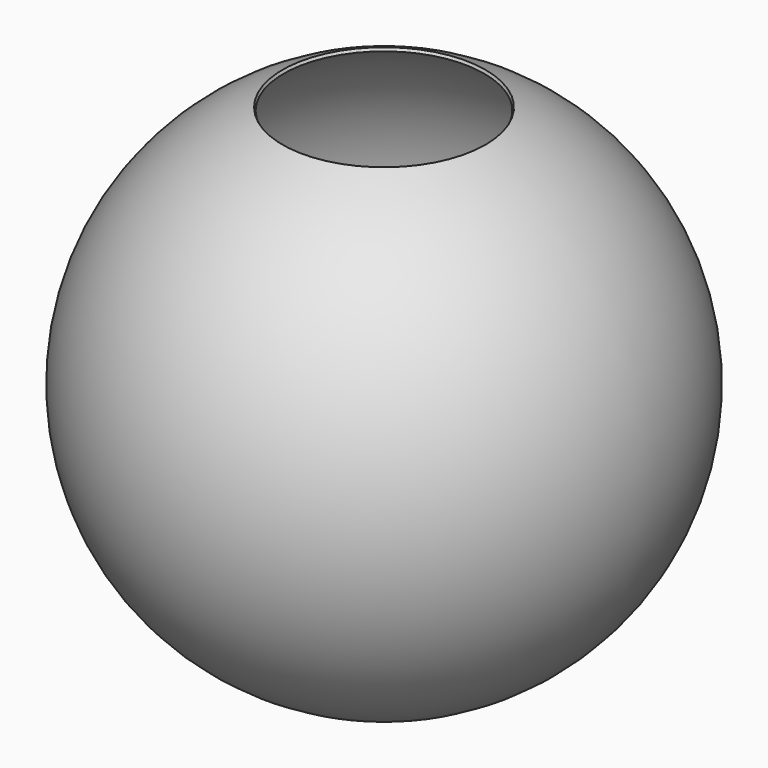
from build123d import *

# Parameters (mm, degrees)
F0_R            = 24
F0_R_2          = 14
F1_DEPTH        = 8
F3_DEPTH        = 1.5
F3_COPIES_COUNT = 5


# Not quite as in the source:
# - a pattern or mirror of a feature is missing from the dataset's text; its kind, count and spacing are read off the source's solid


with BuildPart() as f1:
    # F0 (on Top) → F1 (new body)
    with BuildSketch(Plane.XY):
        Circle(F0_R)
        Circle(F0_R_2, mode=Mode.SUBTRACT)
    extrude(amount=F1_DEPTH)

    # F2 (on Front) → F3 (join, symmetric)
    with BuildSketch(Plane.XZ):
        with BuildLine():
            ThreePointArc((-45.4759894192, -16.4428076923), (-35.9063036344, -5.7161120336), (-22.7166505307, 0))
            Line((-22.7166505307, 0), (-22.7166505307, 8))
            ThreePointArc((-22.7166505307, 8), (-46.7930344517, 15.9905951618), (-64.8907626734, 33.7668182409))
            ThreePointArc((-64.8907626734, 33.7668182409), (-60.6255443353, 6.5576585205), (-45.4759894192, -16.4428076923))
        make_face()
    f3 = extrude(amount=F3_DEPTH, both=True)

    # F3_copies: F3 ×5 about axis
    f3_copies_axis = Axis((0, 0, 0), (0, 0, 1))
    for i in range(1, F3_COPIES_COUNT):
        add(f3.rotate(f3_copies_axis, i * 360 / F3_COPIES_COUNT))


with BuildPart() as f5:
    # F4 (on Front) → F5 (revolve)
    with BuildSketch(Plane.XZ):
        with BuildLine():
            ThreePointArc((25, 90), (65, 30), (25, -30))
            Line((25, -30), (25.3076923077, -30.7384615385))
            ThreePointArc((25.3076923077, -30.7384615385), (65.8, 30), (25.3076923077, 90.7384615385))
            Line((25.3076923077, 90.7384615385), (25, 90))
        make_face()
    revolve(axis=Axis((0, 0, 15), (0, 0, -1)))


solid = Compound([f1.part, f5.part])
